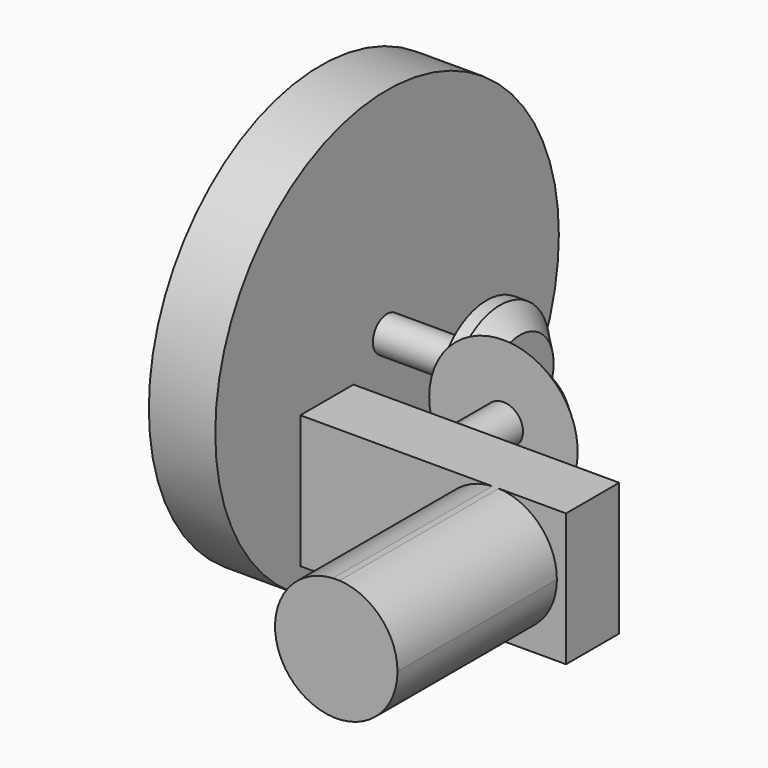
from build123d import *

# Parameters (mm, degrees)
F0_W      = 101.6
F0_H      = 50.8
F1_DEPTH  = 25.4
F3_DEPTH  = 76.2
F4_R      = 7.4724872864
F5_DEPTH  = 50.8
F6_R      = 28.3895179235
F6_R_2    = 7.4724872864
F7_DEPTH  = 6.35
F8_SIZE   = 12.69999
F9_R      = 23.7493356576
F10_DEPTH = 6.35
F11_SIZE  = 7.62
F12_R     = 6.7723102527
F13_DEPTH = 50.8
F14_R     = 82.1200007596
F14_R_2   = 6.7723102527
F15_DEPTH = 12.7


# Not quite as in the source:
# - a fillet or chamfer is up to 0.001 mm smaller than in the source, because OpenCascade refuses the exact size


with BuildPart() as f1:
    # F0 (on Front) → F1 (new body)
    with BuildSketch(Plane.XZ):
        with Locations((50.8, 25.4)):
            Rectangle(F0_W, F0_H)
    extrude(amount=F1_DEPTH)

    # F2 (on face) → F3 (join)
    with BuildSketch(Plane.XZ.offset(25.4)):
        with BuildLine():
            ThreePointArc((73.4443714217, 50.8), (58.5934004133, 10.4401432835), (98.1016742507, 27.4273641407))
            ThreePointArc((98.1016742507, 27.4273641407), (91.6827931143, 43.5295359845), (75.9467730924, 50.8))
            Line((75.9467730924, 50.8), (73.4443714217, 50.8))
        make_face()
    extrude(amount=F3_DEPTH)

    # F4 (on face) → F5 (join)
    with BuildSketch(Plane(origin=(0, 0, 0), x_dir=(-1, 0, 0), z_dir=(0, 1, 0))):
        with Locations((-21.7883531004, 26.4536123723)):
            Circle(F4_R)
    extrude(amount=F5_DEPTH)

    # F6 (on face) → F7 (join, symmetric)
    with BuildSketch(Plane(origin=(0, 50.8, 0), x_dir=(-1, 0, 0), z_dir=(0, 1, 0))):
        with Locations((-21.7883531004, 26.4536123723)):
            Circle(F6_R)
        with Locations((-21.7883531004, 26.4536123723)):
            Circle(F6_R_2, mode=Mode.SUBTRACT)
    extrude(amount=F7_DEPTH, both=True)

    # F8 (size 12.7 in the source; OpenCascade refuses exactly that, so slightly less here)
    f8_edges = [f1.edges().sort_by_distance(p)[0] for p in [
        (50.177871, 57.15, 26.453612),
    ]]
    chamfer(f8_edges, length=F8_SIZE)

    # F9 (on Right) → F10 (join, symmetric)
    with BuildSketch(Plane.YZ):
        with Locations((71.6144831948, 24.2767716783)):
            Circle(F9_R)
    extrude(amount=F10_DEPTH, both=True)

    # F11
    f11_edges = [f1.edges().sort_by_distance(p)[0] for p in [
        (6.35, 79.39333, 46.716034),
        (6.35, 78.162989, 1.448105),
    ]]
    chamfer(f11_edges, length=F11_SIZE)

    # F12 (on face) → F13 (join)
    with BuildSketch(Plane(origin=(-6.35, 0, 0), x_dir=(0, -1, 0), z_dir=(-1, 0, 0))):
        with Locations((-71.6144831948, 24.2767716783)):
            Circle(F12_R)
    extrude(amount=F13_DEPTH)

    # F14 (on face) → F15 (join, symmetric)
    with BuildSketch(Plane(origin=(-57.15, 0, 0), x_dir=(0, -1, 0), z_dir=(-1, 0, 0))):
        with Locations((-71.6144831948, 24.2767716783)):
            Circle(F14_R)
        with Locations((-71.6144831948, 24.2767716783)):
            Circle(F14_R_2, mode=Mode.SUBTRACT)
    extrude(amount=F15_DEPTH, both=True)


solid = f1.part
